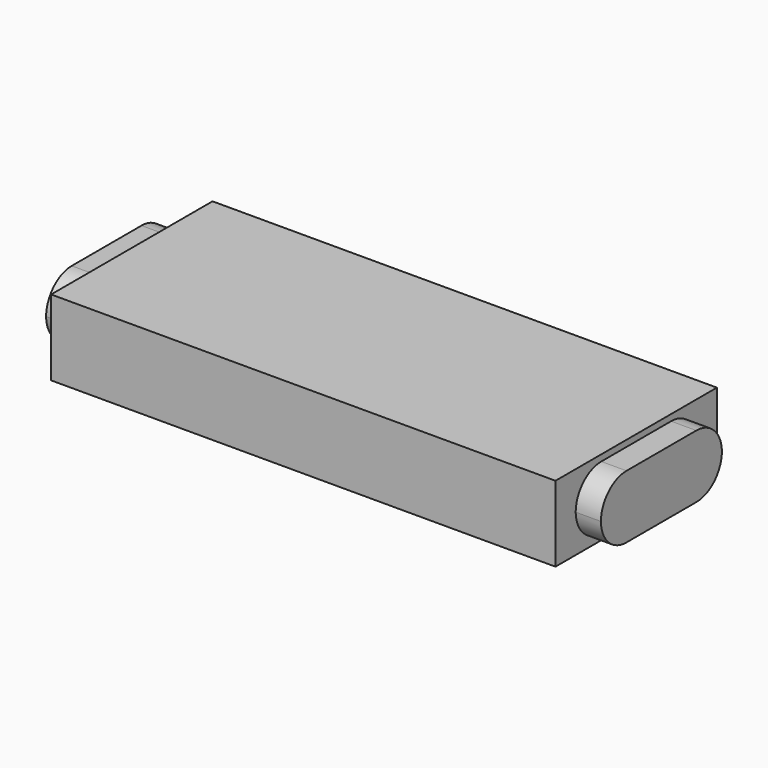
from build123d import *

# Parameters (mm, degrees)
F0_W        = 200
F0_H        = 80
F1_DEPTH    = 30
F2_W        = 60
F2_H        = 25
F3_DEPTH    = 10
F4_W        = 60
F4_H        = 25
F5_DEPTH    = 10
F6_T1_DEPTH = 41.75
F6_T3_DEPTH = 41.75


# Not quite as in the source:
# - a fillet or chamfer that OpenCascade refuses, or shapes differently, is made with other operations: its cross-section is extruded or revolved along the edge and cut away or added


with BuildPart() as f1:
    # F0 (on Top) → F1 (new body)
    with BuildSketch(Plane.XY):
        Rectangle(F0_W, F0_H)
    extrude(amount=F1_DEPTH)

    # F2 (on face) → F3 (join)
    with BuildSketch(Plane(origin=(-100, 0, 0), x_dir=(0, -1, 0), z_dir=(-1, 0, 0))):
        with Locations((0, 15)):
            Rectangle(F2_W, F2_H)
    extrude(amount=F3_DEPTH)

    # F4 (on face) → F5 (join)
    with BuildSketch(Plane.YZ.offset(100)):
        with Locations((0, 15)):
            Rectangle(F4_W, F4_H)
    extrude(amount=F5_DEPTH)

    # F6: fillet of radius 12.7 on 8 edges, made by hand

    # F6_s2 → F6_t1 (cut)
    with BuildSketch(Plane.YZ.offset(100)):
        with BuildLine():
            ThreePointArc((-30, 14.8), (-26.2802561211, 23.7802561211), (-17.3, 27.5))
            Line((-17.3, 27.5), (-30, 27.5))
            Line((-30, 27.5), (-30, 14.8))
        make_face()
        with BuildLine():
            ThreePointArc((-30, 15.2), (-26.2802561211, 6.2197438789), (-17.3, 2.5))
            Line((-17.3, 2.5), (-30, 2.5))
            Line((-30, 2.5), (-30, 15.2))
        make_face()
        with BuildLine():
            ThreePointArc((17.3, 27.5), (26.2802561211, 23.7802561211), (30, 14.8))
            Line((30, 14.8), (30, 27.5))
            Line((30, 27.5), (17.3, 27.5))
        make_face()
        with BuildLine():
            ThreePointArc((30, 15.2), (26.2802561211, 6.2197438789), (17.3, 2.5))
            Line((17.3, 2.5), (30, 2.5))
            Line((30, 2.5), (30, 15.2))
        make_face()
    extrude(amount=F6_T1_DEPTH, mode=Mode.SUBTRACT)

    # F6_s4 → F6_t3 (cut)
    with BuildSketch(Plane.YZ.offset(-141.75)):
        with BuildLine():
            ThreePointArc((30, 14.8), (26.2802561211, 23.7802561211), (17.3, 27.5))
            Line((17.3, 27.5), (30, 27.5))
            Line((30, 27.5), (30, 14.8))
        make_face()
        with BuildLine():
            ThreePointArc((-17.3, 27.5), (-26.2802561211, 23.7802561211), (-30, 14.8))
            Line((-30, 14.8), (-30, 27.5))
            Line((-30, 27.5), (-17.3, 27.5))
        make_face()
        with BuildLine():
            ThreePointArc((-17.3, 2.5), (-26.2802561211, 6.2197438789), (-30, 15.2))
            Line((-30, 15.2), (-30, 2.5))
            Line((-30, 2.5), (-17.3, 2.5))
        make_face()
        with BuildLine():
            ThreePointArc((17.3, 2.5), (26.2802561211, 6.2197438789), (30, 15.2))
            Line((30, 15.2), (30, 2.5))
            Line((30, 2.5), (17.3, 2.5))
        make_face()
    extrude(amount=F6_T3_DEPTH, mode=Mode.SUBTRACT)


solid = f1.part
